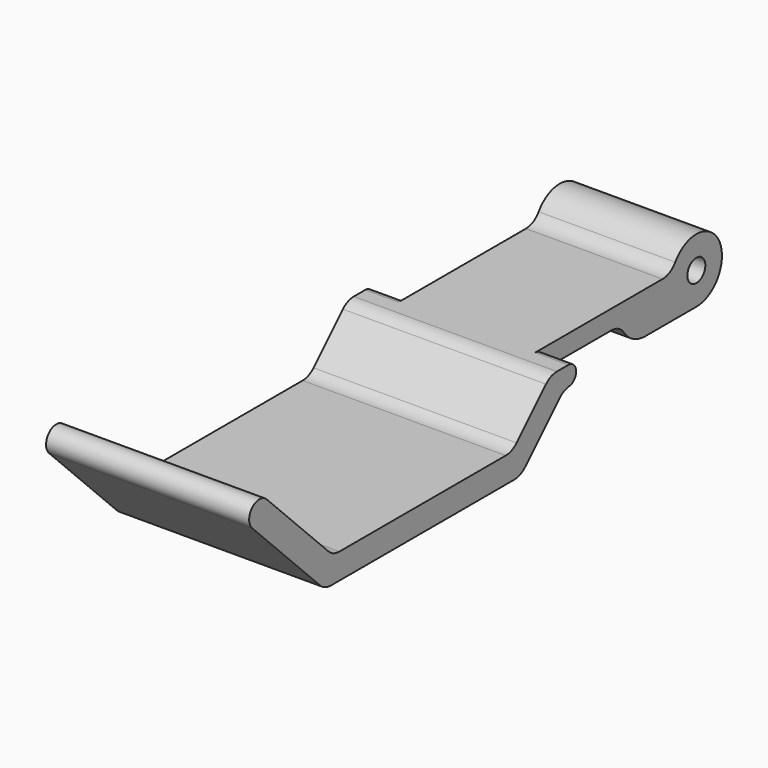
from build123d import *

# Parameters (mm, degrees)
F0_R          = 1.75
F1_DEPTH      = 15.875
F3_DEPTH      = 31.75
F4_R          = 3
F5_W          = 5
F5_H          = 35
F6_DEPTH      = 10.001
F6_DEPTH_BACK = 7.5573491861
F7_T1_DEPTH   = 8.7055800262
F7_T3_DEPTH   = 8.75
F7_T5_DEPTH   = 8.75
F7_T7_DEPTH   = 8.7055800262
F8_DEPTH      = 0.2
F9_DEPTH      = 0.2


# Not quite as in the source:
# - a fillet or chamfer that OpenCascade refuses, or shapes differently, is made with other operations: its cross-section is extruded or revolved along the edge and cut away or added


with BuildPart() as f1:
    # F0 (on Right) → F1 (new body, symmetric)
    with BuildSketch(Plane.YZ):
        with BuildLine():
            Line((-5.2303039929, -1.5), (-4.7696960071, -1.5))
            ThreePointArc((-4.7696960071, -1.5), (5, 0), (-4.7696960071, 1.5))
            Line((-4.7696960071, 1.5), (-35, 1.5))
            Line((-35, 1.5), (-42.5, -6))
            Line((-42.5, -6), (-77.5, -6))
            Line((-77.5, -6), (-90.4705627485, 6.9705627485))
            ThreePointArc((-90.4705627485, 6.9705627485), (-93.2989898732, 6.9705627485), (-93.2989898732, 4.1421356237))
            Line((-93.2989898732, 4.1421356237), (-79.1568542495, -10))
            Line((-79.1568542495, -10), (-40.8431457505, -10))
            Line((-40.8431457505, -10), (-32.3431457505, -1.5))
            Line((-32.3431457505, -1.5), (-14.7696960071, -1.5))
            ThreePointArc((-14.7696960071, -1.5), (-10, -5), (-5.2303039929, -1.5))
        make_face()
        Circle(F0_R, mode=Mode.SUBTRACT)
    extrude(amount=F1_DEPTH, both=True)

    # F2 (on face) → F3 (join, through all)
    with BuildSketch(Plane.YZ.offset(15.875)):
        with BuildLine():
            ThreePointArc((-5.2303039929, -1.5), (-7.0419601085, -4.0311288741), (-10, -5))
            Line((-10, -5), (0, -5))
            ThreePointArc((0, -5), (-2.9580398915, -4.0311288741), (-4.7696960071, -1.5))
            Line((-4.7696960071, -1.5), (-5.2303039929, -1.5))
        make_face()
    extrude(amount=-F3_DEPTH)

    # F4
    f4_edges = [f1.edges().sort_by_distance(p)[0] for p in [
        (0, -4.769696, 1.5),
        (0, -14.769696, -1.5),
        (0, -77.5, -6),
        (0, -79.156854, -10),
        (0, -40.843146, -10),
        (0, -32.343146, -1.5),
        (0, -42.5, -6),
        (0, -35, 1.5),
    ]]
    fillet(f4_edges, radius=F4_R)

    # F5 (on Top) → F6 (cut, two sides)
    with BuildSketch(Plane.XY) as f6_sk:
        with Locations((-13.375, -12.5)):
            Rectangle(F5_W, F5_H)
        with Locations((13.375, -12.5)):
            Rectangle(F5_W, F5_H)
    extrude(amount=-F6_DEPTH, mode=Mode.SUBTRACT)
    extrude(f6_sk.sketch, amount=F6_DEPTH_BACK, mode=Mode.SUBTRACT)

    # F7: fillet of radius 1.5 on 4 edges, made by hand

    # F7_s2 → F7_t1 (cut)
    with BuildSketch(Plane.YZ.offset(10.875)):
        with BuildLine():
            ThreePointArc((-31.3668350211, -1.5118453264), (-30.3932598615, -1.0302531824), (-30, -0.0177679895))
            Line((-30, -0.0177679895), (-29.85, -0.0177679895))
            Line((-29.85, -0.0177679895), (-29.85, -1.5))
            Line((-29.85, -1.5), (-30, -1.65))
            ThreePointArc((-30, -1.65), (-31.1005050634, -1.65), (-31.3535185232, -1.66125306))
            Line((-31.3535185232, -1.66125306), (-31.3668350211, -1.5118453264))
        make_face()
    extrude(amount=F7_T1_DEPTH, mode=Mode.SUBTRACT)

    # F7_s4 → F7_t3 (cut)
    with BuildSketch(Plane.YZ.offset(10.875)):
        with BuildLine():
            ThreePointArc((-30, 0), (-30.4393398282, 1.0606601718), (-31.5, 1.5))
            Line((-31.5, 1.5), (-30, 1.5))
            Line((-30, 1.5), (-30, 0))
        make_face()
    extrude(amount=F7_T3_DEPTH, mode=Mode.SUBTRACT)

    # F7_s6 → F7_t5 (cut)
    with BuildSketch(Plane.YZ.offset(-19.625)):
        with BuildLine():
            ThreePointArc((-30, 0), (-30.4393398282, 1.0606601718), (-31.5, 1.5))
            Line((-31.5, 1.5), (-30, 1.5))
            Line((-30, 1.5), (-30, 0))
        make_face()
    extrude(amount=F7_T5_DEPTH, mode=Mode.SUBTRACT)

    # F7_s8 → F7_t7 (cut)
    with BuildSketch(Plane.YZ.offset(-19.5805800262)):
        with BuildLine():
            ThreePointArc((-31.3668350211, -1.5118453264), (-30.3932598615, -1.0302531824), (-30, -0.0177679895))
            Line((-30, -0.0177679895), (-29.85, -0.0177679895))
            Line((-29.85, -0.0177679895), (-29.85, -1.5))
            Line((-29.85, -1.5), (-30, -1.65))
            ThreePointArc((-30, -1.65), (-31.1005050634, -1.65), (-31.3535185232, -1.66125306))
            Line((-31.3535185232, -1.66125306), (-31.3668350211, -1.5118453264))
        make_face()
    extrude(amount=F7_T7_DEPTH, mode=Mode.SUBTRACT)

    # F8 (cut): a face of the model
    f8_faces = [f1.faces().sort_by_distance(p)[0] for p in [
        (10.875, -9.1101781633, -0.6280033564),
    ]]
    extrude(f8_faces, amount=-F8_DEPTH, mode=Mode.SUBTRACT)

    # F9 (cut): a face of the model
    f9_faces = [f1.faces().sort_by_distance(p)[0] for p in [
        (-10.875, -9.1101781633, -0.6280033564),
    ]]
    extrude(f9_faces, amount=-F9_DEPTH, mode=Mode.SUBTRACT)


solid = f1.part
